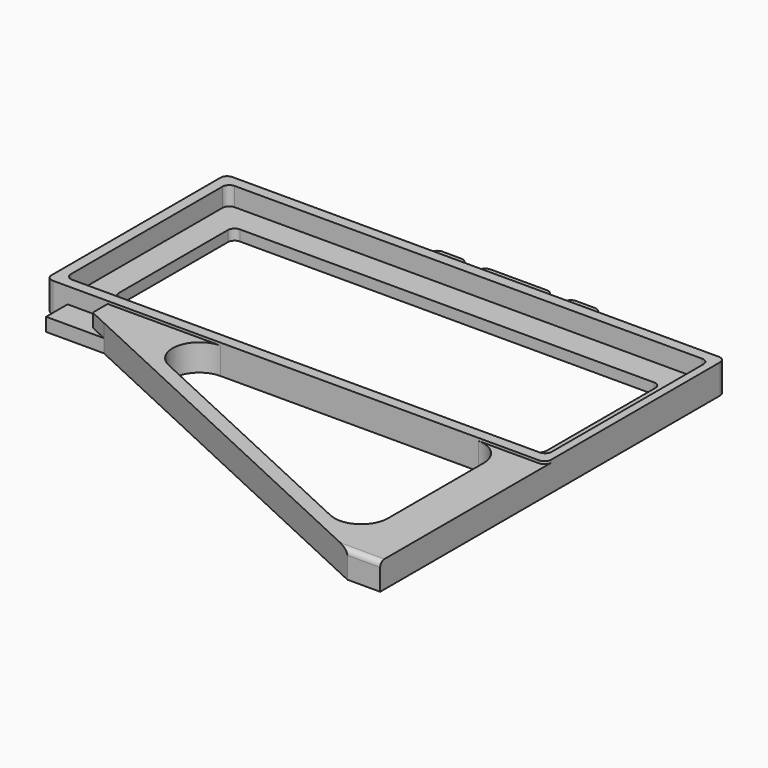
from build123d import *

# Parameters (mm, degrees)
F1_DEPTH = 11
F2_DEPTH = 4
F3_DEPTH = 10
F4_DEPTH = 5
F5_R     = 2


# Not quite as in the source:
# - a feature names something its author has since deleted; it is built from what else it names


with BuildPart() as f1:
    # F0 (on Top) → F1 (new body)
    with BuildSketch(Plane.XY):
        with BuildLine():
            ThreePointArc((93, 77.5), (92.267766953, 79.267766953), (90.5, 80))
            Line((90.5, 80), (37, 80))
            Line((37, 80), (25, 80))
            Line((25, 80), (19, 80))
            Line((19, 80), (-7, 80))
            Line((-7, 80), (-13, 80))
            Line((-13, 80), (-25, 80))
            Line((-25, 80), (-74, 80))
            Line((-74, 80), (-91.5, 80))
            ThreePointArc((-91.5, 80), (-93.267766953, 79.267766953), (-94, 77.5))
            Line((-94, 77.5), (-94, 76))
            Line((-94, 76), (-94, 0))
            Line((-94, 0), (-94, -1.5))
            ThreePointArc((-94, -1.5), (-93.267766953, -3.267766953), (-91.5, -4))
            Line((-91.5, -4), (-88, -4))
            Line((-88, -4), (-86, -4))
            Line((-86, -4), (-71, -4))
            Line((-71, -4), (-28.6959191337, -4))
            Line((-28.6959191337, -4), (67.7072161436, -4))
            Line((67.7072161436, -4), (88, -4))
            Line((88, -4), (90.5, -4))
            ThreePointArc((90.5, -4), (92.267766953, -3.267766953), (93, -1.5))
            Line((93, -1.5), (93, 0))
            Line((93, 0), (93, 76))
            Line((93, 76), (93, 77.5))
        make_face()
        with BuildLine():
            ThreePointArc((90, 2.5), (89.267766953, 0.732233047), (87.5, 0))
            Line((87.5, 0), (-87.5, 0))
            ThreePointArc((-87.5, 0), (-89.267766953, 0.732233047), (-90, 2.5))
            Line((-90, 2.5), (-90, 73.5))
            ThreePointArc((-90, 73.5), (-89.267766953, 75.267766953), (-87.5, 76))
            Line((-87.5, 76), (87.5, 76))
            ThreePointArc((87.5, 76), (89.267766953, 75.267766953), (90, 73.5))
            Line((90, 73.5), (90, 2.5))
        make_face(mode=Mode.SUBTRACT)
    extrude(amount=F1_DEPTH)

    # F0 (on Top) → F2 (join)
    with BuildSketch(Plane.XY):
        with BuildLine():
            Line((-87.5, 0), (87.5, 0))
            ThreePointArc((87.5, 0), (89.267766953, 0.732233047), (90, 2.5))
            Line((90, 2.5), (90, 73.5))
            ThreePointArc((90, 73.5), (89.267766953, 75.267766953), (87.5, 76))
            Line((87.5, 76), (-87.5, 76))
            ThreePointArc((-87.5, 76), (-89.267766953, 75.267766953), (-90, 73.5))
            Line((-90, 73.5), (-90, 2.5))
            ThreePointArc((-90, 2.5), (-89.267766953, 0.732233047), (-87.5, 0))
        make_face()
        with BuildLine():
            Line((-77.5, 66), (77.5, 66))
            ThreePointArc((77.5, 66), (79.267766953, 65.267766953), (80, 63.5))
            Line((80, 63.5), (80, 12.5))
            ThreePointArc((80, 12.5), (79.267766953, 10.732233047), (77.5, 10))
            Line((77.5, 10), (-77.5, 10))
            ThreePointArc((-77.5, 10), (-79.267766953, 10.732233047), (-80, 12.5))
            Line((-80, 12.5), (-80, 63.5))
            ThreePointArc((-80, 63.5), (-79.267766953, 65.267766953), (-77.5, 66))
        make_face(mode=Mode.SUBTRACT)
        with BuildLine():
            Line((-25, 80), (-13, 80))
            Line((-13, 80), (-13, 89.5))
            ThreePointArc((-13, 89.5), (-13.732233047, 91.267766953), (-15.5, 92))
            Line((-15.5, 92), (-22.5, 92))
            ThreePointArc((-22.5, 92), (-24.267766953, 91.267766953), (-25, 89.5))
            Line((-25, 89.5), (-25, 80))
        make_face()
        with BuildLine():
            Line((-7, 80), (19, 80))
            Line((19, 80), (19, 89.5))
            ThreePointArc((19, 89.5), (18.267766953, 91.267766953), (16.5, 92))
            Line((16.5, 92), (-4.5, 92))
            ThreePointArc((-4.5, 92), (-6.267766953, 91.267766953), (-7, 89.5))
            Line((-7, 89.5), (-7, 80))
        make_face()
        with BuildLine():
            Line((25, 80), (37, 80))
            Line((37, 80), (37, 89.5))
            ThreePointArc((37, 89.5), (36.267766953, 91.267766953), (34.5, 92))
            Line((34.5, 92), (27.5, 92))
            ThreePointArc((27.5, 92), (25.732233047, 91.267766953), (25, 89.5))
            Line((25, 89.5), (25, 80))
        make_face()
    extrude(amount=F2_DEPTH)

    # F0 (on Top) → F3 (join)
    with BuildSketch(Plane.XY):
        with BuildLine():
            Line((93, -81.5), (93, -1.5))
            ThreePointArc((93, -1.5), (92.267766953, -3.267766953), (90.5, -4))
            Line((90.5, -4), (88, -4))
            Line((88, -4), (67.7072161436, -4))
            ThreePointArc((67.7072161436, -4), (74.7782839555, -6.9289321881), (77.7072161436, -14))
            Line((77.7072161436, -14), (77.7072161436, -58.7379819401))
            ThreePointArc((77.7072161436, -58.7379819401), (73.0879609173, -67.1669549309), (63.4976990076, -67.8088124137))
            Line((63.4976990076, -67.8088124137), (-32.9054362697, -23.0708304737))
            ThreePointArc((-32.9054362697, -23.0708304737), (-38.4608642113, -11.8445771571), (-28.6959191337, -4))
            Line((-28.6959191337, -4), (-71, -4))
            Line((-71, -4), (-71, -10.9733034172))
            Line((-71, -10.9733034172), (-64.3552474564, -14.0623617917))
            Line((-64.3552474564, -14.0623617917), (80.7072161436, -81.5))
            Line((80.7072161436, -81.5), (93, -81.5))
        make_face()
    extrude(amount=F3_DEPTH)

    # F0 (on Top) → F4 (join)
    with BuildSketch(Plane.XY):
        Polygon((-71, -14.0623617917), (-71, -10.9733034172), (-86, -4), (-86, -14.0623617917), align=None)
        Polygon((-86, -4), (-71, -10.9733034172), (-71, -4), align=None)
        Polygon((-71, -14.0623617917), (-64.3552474564, -14.0623617917), (-71, -10.9733034172), align=None)
    extrude(amount=F4_DEPTH)

    # F5
    f5_edges = [f1.edges().sort_by_distance(p)[0] for p in [
        (86.853608, -81.5, 10),
    ]]
    fillet(f5_edges, radius=F5_R)


solid = f1.part
